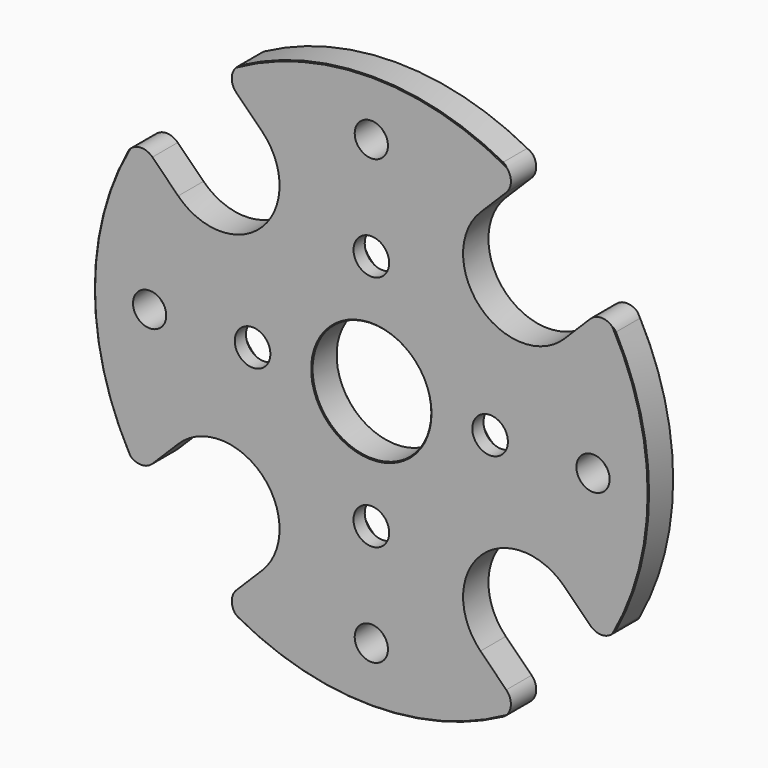
from build123d import *

# Parameters (mm, degrees)
F0_R           = 35
F0_R_2         = 7.5
F1_DEPTH       = 4
F2_SIZE        = 0.1
F4_D           = 4.5
F4_CSINK_D     = 8.96
F4_CSINK_ANGLE = 90
F6_DEPTH       = 4
F7_R           = 2
F9_D           = 4.2


# Not quite as in the source:
# - a feature names something its author has since deleted; it is built from what else it names


with BuildPart() as f1:
    # F0 (on Front) → F1 (new body)
    with BuildSketch(Plane.XZ):
        Circle(F0_R)
        Circle(F0_R_2, mode=Mode.SUBTRACT)
    extrude(amount=F1_DEPTH)

    # F2
    f2_edges = [f1.edges().sort_by_distance(p)[0] for p in [
        (-35, -4, 0),
        (-35, 0, 0),
        (-7.5, 0, 0),
        (-7.5, -4, 0),
    ]]
    chamfer(f2_edges, length=F2_SIZE)

    # F4 (through all)
    with Locations(Plane(origin=(0, 0, 0), x_dir=(1, 0, 0), z_dir=(0, 1, 0))):
        with Locations((-15, 0), (0, 15), (15, 0), (0, -15)):
            CounterSinkHole(F4_D / 2, F4_CSINK_D / 2, counter_sink_angle=F4_CSINK_ANGLE)

    # F5 (on face) → F6 (cut, through all)
    with BuildSketch(Plane(origin=(0, 0, 0), x_dir=(-1, 0, 0), z_dir=(0, 1, 0))):
        with BuildLine():
            Line((-25.2671224679, -35.8737241857), (-13.7885822331, -24.3951839509))
            ThreePointArc((-13.7885822331, -24.3951839509), (-13.7885822331, -13.7885822331), (-24.3951839509, -13.7885822331))
            Line((-24.3951839509, -13.7885822331), (-35.8737241857, -25.2671224679))
            Line((-35.8737241857, -25.2671224679), (-25.2671224679, -35.8737241857))
        make_face()
        with BuildLine():
            Line((13.7885822331, -24.3951839509), (25.2671224679, -35.8737241857))
            Line((25.2671224679, -35.8737241857), (35.8737241857, -25.2671224679))
            Line((35.8737241857, -25.2671224679), (24.3951839509, -13.7885822331))
            ThreePointArc((24.3951839509, -13.7885822331), (13.7885822331, -13.7885822331), (13.7885822331, -24.3951839509))
        make_face()
        with BuildLine():
            Line((24.3951839509, 13.7885822331), (35.8737241857, 25.2671224679))
            Line((35.8737241857, 25.2671224679), (25.2671224679, 35.8737241857))
            Line((25.2671224679, 35.8737241857), (13.7885822331, 24.3951839509))
            ThreePointArc((13.7885822331, 24.3951839509), (13.7885822331, 13.7885822331), (24.3951839509, 13.7885822331))
        make_face()
        with BuildLine():
            Line((-13.7885822331, 24.3951839509), (-25.2671224679, 35.8737241857))
            Line((-25.2671224679, 35.8737241857), (-35.8737241857, 25.2671224679))
            Line((-35.8737241857, 25.2671224679), (-24.3951839509, 13.7885822331))
            ThreePointArc((-24.3951839509, 13.7885822331), (-13.7885822331, 13.7885822331), (-13.7885822331, 24.3951839509))
        make_face()
    extrude(amount=-F6_DEPTH, mode=Mode.SUBTRACT)

    # F7
    f7_edges = [f1.edges().sort_by_distance(p)[0] for p in [
        (29.47715, -2, -18.870549),
        (18.870549, -2, -29.47715),
        (-18.870549, -2, -29.47715),
        (-29.47715, -2, -18.870549),
        (-29.47715, -2, 18.870549),
        (-18.870549, -2, 29.47715),
        (18.870549, -2, 29.47715),
        (29.47715, -2, 18.870549),
    ]]
    fillet(f7_edges, radius=F7_R)

    # F9 (through all)
    with Locations(Plane.XZ.offset(4)):
        with Locations((0, 28), (28, 0), (0, -28), (-28, 0)):
            Hole(F9_D / 2)


solid = f1.part
